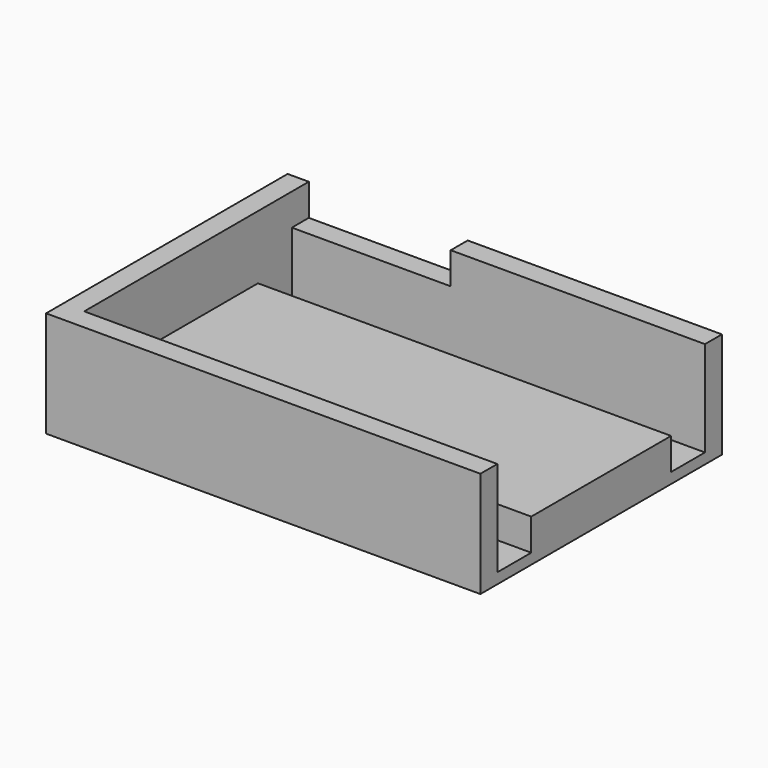
from build123d import *

# Parameters (mm, degrees)
F1_DEPTH = 1
F0_W     = 39
F0_H     = 4
F0_H_2   = 16.5
F2_DEPTH = 4
F0_W_2   = 15
F0_H_3   = 2
F3_DEPTH = 7
F0_W_3   = 24
F4_DEPTH = 10


# Not quite as in the source:
# - a feature names something its author has since deleted; it is built from what else it names


with BuildPart() as f1:
    # F0 (on Top) → F1 (new body)
    with BuildSketch(Plane.XY):
        Polygon((17, 26.5), (2, 26.5), (2, 22.5), (41, 22.5), (41, 26.5), align=None)
    extrude(amount=F1_DEPTH)



with BuildPart() as f1b:
    # F0 (on Top) → F1, piece 2 (new body)
    with BuildSketch(Plane.XY):
        with Locations((21.5, 4)):
            Rectangle(F0_W, F0_H)
    extrude(amount=F1_DEPTH)


with BuildPart() as f1_1:
    add(f1.part)

    add(f1b.part)  # F2 merges F1b
    # F0 (on Top) → F2 (join)
    with BuildSketch(Plane.XY):
        with Locations((21.5, 14.25)):
            Rectangle(F0_W, F0_H_2)
    extrude(amount=F2_DEPTH)

    # F0 (on Top) → F3 (join)
    with BuildSketch(Plane.XY):
        with Locations((9.5, 27.5)):
            Rectangle(F0_W_2, F0_H_3)
    extrude(amount=F3_DEPTH)

    # F0 (on Top) → F4 (join)
    with BuildSketch(Plane.XY):
        with Locations((29, 27.5)):
            Rectangle(F0_W_3, F0_H_3)
        Polygon((2, 22.5), (2, 26.5), (2, 28.5), (0, 28.5), (0, 2), (2, 2), (2, 6), align=None)
        Polygon((41, 2), (2, 2), (0, 2), (0, 0), (41, 0), align=None)
    extrude(amount=F4_DEPTH)


solid = f1_1.part
